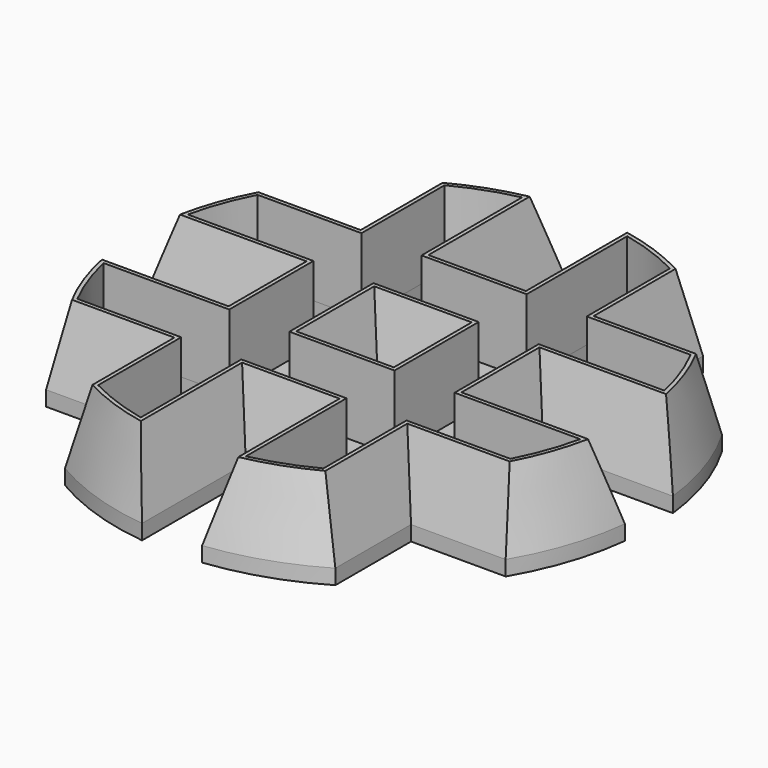
from build123d import *

# Parameters (mm, degrees)
F0_W     = 14
F0_H     = 14
F0_W_2   = 8
F0_H_2   = 8
F1_DEPTH = 10
F2_SIZE2 = 2.49327
F2_SIZE  = 9.99999
F3_SIZE2 = 2.49327
F3_SIZE  = 9.99999
F4_W     = 8
F4_H     = 8
F5_DEPTH = 2


# Not quite as in the source:
# - a fillet or chamfer is up to 0.001 mm smaller than in the source, because OpenCascade refuses the exact size
# - a feature names something its author has since deleted; it is built from what else it names


with BuildPart() as f1:
    # F0 (on Top) → F1 (new body)
    with BuildSketch(Plane.XY):
        Rectangle(F0_W, F0_H)
        Rectangle(F0_W_2, F0_H_2, mode=Mode.SUBTRACT)
    extrude(amount=F1_DEPTH)

    # F3 (size 10 and 2.4932800284 in the source; OpenCascade refuses exactly that, so slightly less here)
    f3_edges = [f1.edges().sort_by_distance(p)[0] for p in [
        (4, 0, 10),
        (0, -4, 10),
        (-4, 0, 10),
        (0, 4, 10),
    ]]
    chamfer(f3_edges, length=F3_SIZE, length2=F3_SIZE2)


with BuildPart() as f1b:
    # F0 (on Top) → F1, piece 2 (new body)
    with BuildSketch(Plane.XY):
        with BuildLine():
            ThreePointArc((-30.5982025616, 18), (-33.6717151002, 11.2456926069), (-35.2739280489, 4))
            Line((-35.2739280489, 4), (-18, 4))
            Line((-18, 4), (-18, -4))
            Line((-18, -4), (-35.2739280489, -4))
            ThreePointArc((-35.2739280489, -4), (-33.6717151002, -11.2456926069), (-30.5982025616, -18))
            Line((-30.5982025616, -18), (-18, -18))
            Line((-18, -18), (-18, -30.5982025616))
            ThreePointArc((-18, -30.5982025616), (-11.2456926069, -33.6717151002), (-4, -35.2739280489))
            Line((-4, -35.2739280489), (-4, -18))
            Line((-4, -18), (4, -18))
            Line((4, -18), (4, -35.2739280489))
            ThreePointArc((4, -35.2739280489), (11.2456926069, -33.6717151002), (18, -30.5982025616))
            Line((18, -30.5982025616), (18, -18))
            Line((18, -18), (30.5982025616, -18))
            ThreePointArc((30.5982025616, -18), (33.6717151002, -11.2456926069), (35.2739280489, -4))
            Line((35.2739280489, -4), (18, -4))
            Line((18, -4), (18, 4))
            Line((18, 4), (35.2739280489, 4))
            ThreePointArc((35.2739280489, 4), (33.6717151002, 11.2456926069), (30.5982025616, 18))
            Line((30.5982025616, 18), (18, 18))
            Line((18, 18), (18, 30.5982025616))
            ThreePointArc((18, 30.5982025616), (11.2456926069, 33.6717151002), (4, 35.2739280489))
            Line((4, 35.2739280489), (4, 18))
            Line((4, 18), (-4, 18))
            Line((-4, 18), (-4, 35.2739280489))
            ThreePointArc((-4, 35.2739280489), (-11.2456926069, 33.6717151002), (-18, 30.5982025616))
            Line((-18, 30.5982025616), (-18, 18))
            Line((-18, 18), (-30.5982025616, 18))
        make_face()
        with BuildLine():
            ThreePointArc((-31.7372021451, 7), (-30.5473253804, 11.0955356834), (-28.8314064867, 15))
            Line((-28.8314064867, 15), (-15, 15))
            Line((-15, 15), (-15, 28.8314064867))
            ThreePointArc((-15, 28.8314064867), (-11.0955356834, 30.5473253804), (-7, 31.7372021451))
            Line((-7, 31.7372021451), (-7, 15))
            Line((-7, 15), (7, 15))
            Line((7, 15), (7, 31.7372021451))
            ThreePointArc((7, 31.7372021451), (11.0955356834, 30.5473253804), (15, 28.8314064867))
            Line((15, 28.8314064867), (15, 15))
            Line((15, 15), (28.8314064867, 15))
            ThreePointArc((28.8314064867, 15), (30.5473253804, 11.0955356834), (31.7372021451, 7))
            Line((31.7372021451, 7), (15, 7))
            Line((15, 7), (15, -7))
            Line((15, -7), (31.7372021451, -7))
            ThreePointArc((31.7372021451, -7), (30.5473253804, -11.0955356834), (28.8314064867, -15))
            Line((28.8314064867, -15), (15, -15))
            Line((15, -15), (15, -28.8314064867))
            ThreePointArc((15, -28.8314064867), (11.0955356834, -30.5473253804), (7, -31.7372021451))
            Line((7, -31.7372021451), (7, -15))
            Line((7, -15), (-7, -15))
            Line((-7, -15), (-7, -31.7372021451))
            ThreePointArc((-7, -31.7372021451), (-11.0955356834, -30.5473253804), (-15, -28.8314064867))
            Line((-15, -28.8314064867), (-15, -15))
            Line((-15, -15), (-28.8314064867, -15))
            ThreePointArc((-28.8314064867, -15), (-30.5473253804, -11.0955356834), (-31.7372021451, -7))
            Line((-31.7372021451, -7), (-15, -7))
            Line((-15, -7), (-15, 7))
            Line((-15, 7), (-31.7372021451, 7))
        make_face(mode=Mode.SUBTRACT)
    extrude(amount=F1_DEPTH)

    # F2 (size 10 and 2.4932800284 in the source; OpenCascade refuses exactly that, so slightly less here)
    f2_edges = [f1b.edges().sort_by_distance(p)[0] for p in [
        (26.636964, -4, 10),
        (33.671715, -11.245693, 10),
        (24.299101, -18, 10),
        (18, -24.299101, 10),
        (11.245693, -33.671715, 10),
        (4, -26.636964, 10),
        (-4, -26.636964, 10),
        (-11.245693, -33.671715, 10),
        (-18, -24.299101, 10),
        (-24.299101, -18, 10),
        (-33.671715, -11.245693, 10),
        (-26.636964, -4, 10),
        (-18, 0, 10),
        (-26.636964, 4, 10),
        (-33.671715, 11.245693, 10),
        (-24.299101, 18, 10),
        (-18, 24.299101, 10),
        (-11.245693, 33.671715, 10),
        (-4, 26.636964, 10),
        (0, 18, 10),
        (4, 26.636964, 10),
        (11.245693, 33.671715, 10),
        (18, 24.299101, 10),
        (24.299101, 18, 10),
        (33.671715, 11.245693, 10),
        (26.636964, 4, 10),
        (18, 0, 10),
        (0, -18, 10),
    ]]
    chamfer(f2_edges, length=F2_SIZE, length2=F2_SIZE2)


with BuildPart() as f5:
    # F4 (on face) → F5 (new body)
    with BuildSketch(Plane.XY):
        with BuildLine():
            Line((-35.2739280489, 4), (-18, 4))
            Line((-18, 4), (-18, -4))
            Line((-18, -4), (-35.2739280489, -4))
            ThreePointArc((-35.2739280489, -4), (-33.6717151002, -11.2456926069), (-30.5982025616, -18))
            Line((-30.5982025616, -18), (-18, -18))
            Line((-18, -18), (-18, -30.5982025616))
            ThreePointArc((-18, -30.5982025616), (-11.2456926069, -33.6717151002), (-4, -35.2739280489))
            Line((-4, -35.2739280489), (-4, -18))
            Line((-4, -18), (4, -18))
            Line((4, -18), (4, -35.2739280489))
            ThreePointArc((4, -35.2739280489), (11.2456926069, -33.6717151002), (18, -30.5982025616))
            Line((18, -30.5982025616), (18, -18))
            Line((18, -18), (30.5982025616, -18))
            ThreePointArc((30.5982025616, -18), (33.6717151002, -11.2456926069), (35.2739280489, -4))
            Line((35.2739280489, -4), (18, -4))
            Line((18, -4), (18, 4))
            Line((18, 4), (35.2739280489, 4))
            ThreePointArc((35.2739280489, 4), (33.6717151002, 11.2456926069), (30.5982025616, 18))
            Line((30.5982025616, 18), (18, 18))
            Line((18, 18), (18, 30.5982025616))
            ThreePointArc((18, 30.5982025616), (11.2456926069, 33.6717151002), (4, 35.2739280489))
            Line((4, 35.2739280489), (4, 18))
            Line((4, 18), (-4, 18))
            Line((-4, 18), (-4, 35.2739280489))
            ThreePointArc((-4, 35.2739280489), (-11.2456926069, 33.6717151002), (-18, 30.5982025616))
            Line((-18, 30.5982025616), (-18, 18))
            Line((-18, 18), (-30.5982025616, 18))
            ThreePointArc((-30.5982025616, 18), (-33.6717151002, 11.2456926069), (-35.2739280489, 4))
        make_face()
        with BuildLine():
            ThreePointArc((-15, 28.8314064867), (-11.0955356834, 30.5473253804), (-7, 31.7372021451))
            Line((-7, 31.7372021451), (-7, 15))
            Line((-7, 15), (7, 15))
            Line((7, 15), (7, 31.7372021451))
            ThreePointArc((7, 31.7372021451), (11.0955356834, 30.5473253804), (15, 28.8314064867))
            Line((15, 28.8314064867), (15, 15))
            Line((15, 15), (28.8314064867, 15))
            ThreePointArc((28.8314064867, 15), (30.5473253804, 11.0955356834), (31.7372021451, 7))
            Line((31.7372021451, 7), (15, 7))
            Line((15, 7), (15, -7))
            Line((15, -7), (31.7372021451, -7))
            ThreePointArc((31.7372021451, -7), (30.5473253804, -11.0955356834), (28.8314064867, -15))
            Line((28.8314064867, -15), (15, -15))
            Line((15, -15), (15, -28.8314064867))
            ThreePointArc((15, -28.8314064867), (11.0955356834, -30.5473253804), (7, -31.7372021451))
            Line((7, -31.7372021451), (7, -15))
            Line((7, -15), (-7, -15))
            Line((-7, -15), (-7, -31.7372021451))
            ThreePointArc((-7, -31.7372021451), (-11.0955356834, -30.5473253804), (-15, -28.8314064867))
            Line((-15, -28.8314064867), (-15, -15))
            Line((-15, -15), (-28.8314064867, -15))
            ThreePointArc((-28.8314064867, -15), (-30.5473253804, -11.0955356834), (-31.7372021451, -7))
            Line((-31.7372021451, -7), (-15, -7))
            Line((-15, -7), (-15, 7))
            Line((-15, 7), (-31.7372021451, 7))
            ThreePointArc((-31.7372021451, 7), (-30.5473253804, 11.0955356834), (-28.8314064867, 15))
            Line((-28.8314064867, 15), (-15, 15))
            Line((-15, 15), (-15, 28.8314064867))
        make_face(mode=Mode.SUBTRACT)
        Polygon((7, 15), (-7, 15), (-7, 7), (-15, 7), (-15, -7), (-7, -7), (-7, -15), (7, -15), (7, -7), (15, -7), (15, 7), (7, 7), align=None)
        Rectangle(F4_W, F4_H, mode=Mode.SUBTRACT)
    extrude(amount=-F5_DEPTH)


solid = Compound([f1.part, f1b.part, f5.part])
